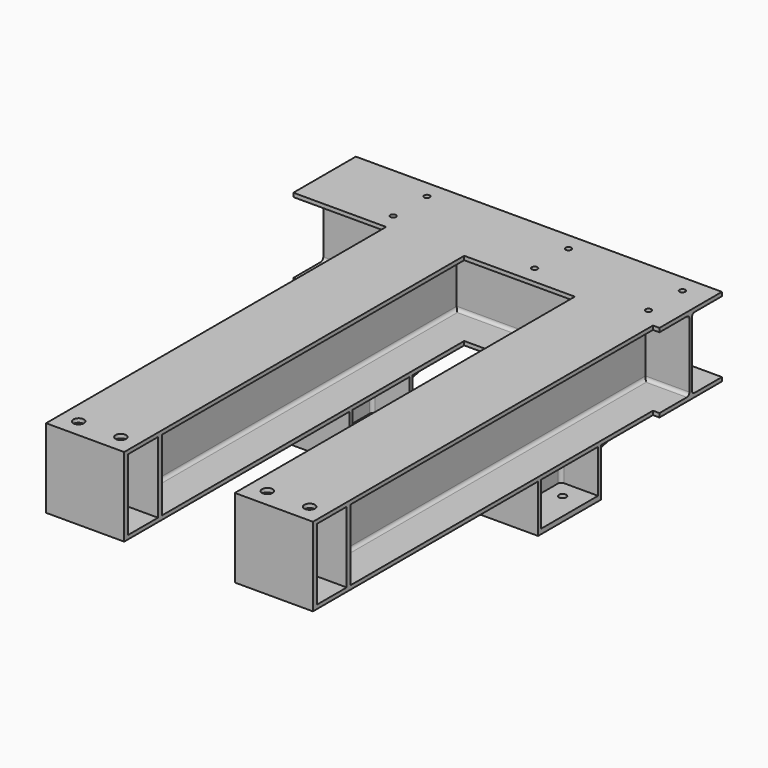
from build123d import *

# Parameters (mm, degrees)
F1_DEPTH  = 714.375
F3_D      = 22.225
F3_DEPTH  = 76.2
F3_TIP    = 6.6770636289
F5_DEPTH  = 1792.224
F6_W      = 304.8
F6_H      = 307.975
F7_DEPTH  = 19.05
F10_D     = 22.225
F10_DEPTH = 76.2
F10_TIP   = 6.6770636289
F11_W     = 19.05
F11_H     = 277.495
F12_DEPTH = 304.8
F13_W     = 19.05
F13_H     = 277.495
F14_DEPTH = 304.8
F16_D     = 41.402
F18_DEPTH = 168.402
F19_W     = 304.8
F19_H     = 307.848
F20_DEPTH = 19.05
F22_D     = 28.448
F22_2_D   = 28.448
F24_W     = 19.05
F24_H     = 457.2
F25_DEPTH = 168.402
F27_DEPTH = 1260.349


# Not quite as in the source:
# - a length typed as a fraction of an inch, garbled in the dataset ("3 / 203.2 mm" for 3/8 in), is restored


with BuildPart() as f1:
    # F0 (on Right) → F1 (new body, symmetric)
    with BuildSketch(Plane.YZ):
        with BuildLine():
            Line((152.4, 153.9875), (-152.4, 153.9875))
            Line((-152.4, 153.9875), (-152.4, 138.7475))
            Line((-152.4, 138.7475), (-19.05, 138.7475))
            ThreePointArc((-19.05, 138.7475), (-10.0697438789, 135.0277561211), (-6.35, 126.0475))
            Line((-6.35, 126.0475), (-6.35, -126.0475))
            ThreePointArc((-6.35, -126.0475), (-10.0697438789, -135.0277561211), (-19.05, -138.7475))
            Line((-19.05, -138.7475), (-152.4, -138.7475))
            Line((-152.4, -138.7475), (-152.4, -153.9875))
            Line((-152.4, -153.9875), (152.4, -153.9875))
            Line((152.4, -153.9875), (152.4, -138.7475))
            Line((152.4, -138.7475), (19.05, -138.7475))
            ThreePointArc((19.05, -138.7475), (10.0697438789, -135.0277561211), (6.35, -126.0475))
            Line((6.35, -126.0475), (6.35, 126.0475))
            ThreePointArc((6.35, 126.0475), (10.0697438789, 135.0277561211), (19.05, 138.7475))
            Line((19.05, 138.7475), (152.4, 138.7475))
            Line((152.4, 138.7475), (152.4, 153.9875))
        make_face()
    extrude(amount=F1_DEPTH, both=True)

    # F3
    with Locations(Plane.XY.offset(153.9875)):
        with Locations((-381, 82.55), (-381, -82.55), (171.45, 82.55), (171.45, -82.55), (615.95, 82.55), (615.95, -82.55)):
            Hole(F3_D / 2, depth=F3_DEPTH)
            with Locations((0, 0, -(F3_DEPTH + F3_TIP / 2))):  # 118° drill point
                Cone(0, F3_D / 2, F3_TIP, mode=Mode.SUBTRACT)


with BuildPart() as f5:
    # F4 (on Front) → F5 (new body)
    with BuildSketch(Plane.XZ):
        with BuildLine():
            Line((-47.625, 153.9875), (-352.425, 153.9875))
            Line((-352.425, 153.9875), (-352.425, 138.7475))
            Line((-352.425, 138.7475), (-219.075, 138.7475))
            ThreePointArc((-219.075, 138.7475), (-210.0947438789, 135.0277561211), (-206.375, 126.0475))
            Line((-206.375, 126.0475), (-206.375, -126.0475))
            ThreePointArc((-206.375, -126.0475), (-210.0947438789, -135.0277561211), (-219.075, -138.7475))
            Line((-219.075, -138.7475), (-352.425, -138.7475))
            Line((-352.425, -138.7475), (-352.425, -153.9875))
            Line((-352.425, -153.9875), (-47.625, -153.9875))
            Line((-47.625, -153.9875), (-47.625, -138.7475))
            Line((-47.625, -138.7475), (-180.975, -138.7475))
            ThreePointArc((-180.975, -138.7475), (-189.9552561211, -135.0277561211), (-193.675, -126.0475))
            Line((-193.675, -126.0475), (-193.675, 126.0475))
            ThreePointArc((-193.675, 126.0475), (-189.9552561211, 135.0277561211), (-180.975, 138.7475))
            Line((-180.975, 138.7475), (-47.625, 138.7475))
            Line((-47.625, 138.7475), (-47.625, 153.9875))
        make_face()
    extrude(amount=F5_DEPTH)


with BuildPart() as f5b:
    # F4 (on Front) → F5, piece 2 (new body)
    with BuildSketch(Plane.XZ):
        with BuildLine():
            Line((688.975, 153.9875), (384.175, 153.9875))
            Line((384.175, 153.9875), (384.175, 138.7475))
            Line((384.175, 138.7475), (517.525, 138.7475))
            ThreePointArc((517.525, 138.7475), (526.5052561211, 135.0277561211), (530.225, 126.0475))
            Line((530.225, 126.0475), (530.225, -126.0475))
            ThreePointArc((530.225, -126.0475), (526.5052561211, -135.0277561211), (517.525, -138.7475))
            Line((517.525, -138.7475), (384.175, -138.7475))
            Line((384.175, -138.7475), (384.175, -153.9875))
            Line((384.175, -153.9875), (688.975, -153.9875))
            Line((688.975, -153.9875), (688.975, -138.7475))
            Line((688.975, -138.7475), (555.625, -138.7475))
            ThreePointArc((555.625, -138.7475), (546.6447438789, -135.0277561211), (542.925, -126.0475))
            Line((542.925, -126.0475), (542.925, 126.0475))
            ThreePointArc((542.925, 126.0475), (546.6447438789, 135.0277561211), (555.625, 138.7475))
            Line((555.625, 138.7475), (688.975, 138.7475))
            Line((688.975, 138.7475), (688.975, 153.9875))
        make_face()
    extrude(amount=F5_DEPTH)


with BuildPart() as f7:
    # F6 (on face) → F7 (new body)
    with BuildSketch(Plane.XZ.offset(1792.224)):
        with Locations((-200.025, 0)):
            Rectangle(F6_W, F6_H)
    extrude(amount=F7_DEPTH)


with BuildPart() as f7b:
    # F6 (on face) → F7, piece 2 (new body)
    with BuildSketch(Plane.XZ.offset(1792.224)):
        with Locations((536.575, 0)):
            Rectangle(F6_W, F6_H)
    extrude(amount=F7_DEPTH)


with BuildPart() as f1_1:
    add(f1.part)

    # F8: union F5, F5b, F7b, F7
    add(f5.part)
    add(f5b.part)
    add(f7b.part)
    add(f7.part)

    # F10
    with Locations(Plane.XY.offset(153.9875)):
        with Locations((615.95, -82.55)):
            Hole(F10_D / 2, depth=F10_DEPTH)
            with Locations((0, 0, -(F10_DEPTH + F10_TIP / 2))):  # 118° drill point
                Cone(0, F10_D / 2, F10_TIP, mode=Mode.SUBTRACT)

    # F11 (on face) → F12 (join)
    with BuildSketch(Plane.YZ.offset(688.975)):
        with Locations((-1636.649, 0)):
            Rectangle(F11_W, F11_H)
    extrude(amount=-F12_DEPTH)

    # F13 (on face) → F14 (join)
    with BuildSketch(Plane(origin=(-352.425, 0, 0), x_dir=(0, -1, 0), z_dir=(-1, 0, 0))):
        with Locations((1636.649, 0)):
            Rectangle(F13_W, F13_H)
    extrude(amount=-F14_DEPTH)

    # F16 (through all)
    with Locations(Plane.XY.offset(153.9875)):
        with Locations((619.125, -1739.9), (454.025, -1739.9), (-117.475, -1739.9), (-282.575, -1739.9)):
            Hole(F16_D / 2)


with BuildPart() as f18:
    # F17 (on face) → F18 (new body)
    with BuildSketch(Plane(origin=(0, 0, -153.9875), x_dir=(1, 0, 0), z_dir=(0, 0, -1))):
        with BuildLine():
            Line((-352.425, 420.116), (-352.425, 404.876))
            Line((-352.425, 404.876), (-47.625, 404.876))
            Line((-47.625, 404.876), (-47.625, 420.116))
            Line((-47.625, 420.116), (-180.975, 420.116))
            ThreePointArc((-180.975, 420.116), (-189.9552561211, 423.8357438789), (-193.675, 432.816))
            Line((-193.675, 432.816), (-193.675, 684.784))
            ThreePointArc((-193.675, 684.784), (-189.9552561211, 693.7642561211), (-180.975, 697.484))
            Line((-180.975, 697.484), (-47.625, 697.484))
            Line((-47.625, 697.484), (-47.625, 712.724))
            Line((-47.625, 712.724), (-352.425, 712.724))
            Line((-352.425, 712.724), (-352.425, 697.484))
            Line((-352.425, 697.484), (-219.075, 697.484))
            ThreePointArc((-219.075, 697.484), (-210.0947438789, 693.7642561211), (-206.375, 684.784))
            Line((-206.375, 684.784), (-206.375, 432.816))
            ThreePointArc((-206.375, 432.816), (-210.0947438789, 423.8357438789), (-219.075, 420.116))
            Line((-219.075, 420.116), (-352.425, 420.116))
        make_face()
    extrude(amount=F18_DEPTH)


with BuildPart() as f18b:
    # F17 (on face) → F18, piece 2 (new body)
    with BuildSketch(Plane(origin=(0, 0, -153.9875), x_dir=(1, 0, 0), z_dir=(0, 0, -1))):
        with BuildLine():
            Line((688.975, 420.116), (555.625, 420.116))
            ThreePointArc((555.625, 420.116), (546.6447438789, 423.8357438789), (542.925, 432.816))
            Line((542.925, 432.816), (542.925, 684.784))
            ThreePointArc((542.925, 684.784), (546.6447438789, 693.7642561211), (555.625, 697.484))
            Line((555.625, 697.484), (688.975, 697.484))
            Line((688.975, 697.484), (688.975, 712.724))
            Line((688.975, 712.724), (384.175, 712.724))
            Line((384.175, 712.724), (384.175, 697.484))
            Line((384.175, 697.484), (517.525, 697.484))
            ThreePointArc((517.525, 697.484), (526.5052561211, 693.7642561211), (530.225, 684.784))
            Line((530.225, 684.784), (530.225, 432.816))
            ThreePointArc((530.225, 432.816), (526.5052561211, 423.8357438789), (517.525, 420.116))
            Line((517.525, 420.116), (384.175, 420.116))
            Line((384.175, 420.116), (384.175, 404.876))
            Line((384.175, 404.876), (688.975, 404.876))
            Line((688.975, 404.876), (688.975, 420.116))
        make_face()
    extrude(amount=F18_DEPTH)


with BuildPart() as f20:
    # F19 (on face) → F20 (new body)
    with BuildSketch(Plane(origin=(0, 0, -322.3895), x_dir=(1, 0, 0), z_dir=(0, 0, -1))):
        with Locations((-200.025, 558.8)):
            Rectangle(F19_W, F19_H)
    extrude(amount=F20_DEPTH)

    # F22 (through all)
    with Locations(Plane(origin=(0, 0, -341.4395), x_dir=(1, 0, 0), z_dir=(0, 0, -1))):
        with Locations((-269.1834158416, 628.65), (-130.8665841584, 628.65), (-269.1834158416, 488.95), (-130.8665841584, 488.95), (467.4165841584, 628.65), (605.7334158416, 628.65), (605.7334158416, 488.95), (467.4165841584, 488.95)):
            Hole(F22_D / 2)


with BuildPart() as f20b:
    # F19 (on face) → F20, piece 2 (new body)
    with BuildSketch(Plane(origin=(0, 0, -322.3895), x_dir=(1, 0, 0), z_dir=(0, 0, -1))):
        with Locations((536.575, 558.8)):
            Rectangle(F19_W, F19_H)
    extrude(amount=F20_DEPTH)

    # F22#2 (through all)
    with Locations(Plane(origin=(0, 0, -341.4395), x_dir=(1, 0, 0), z_dir=(0, 0, -1))):
        with Locations((-269.1834158416, 628.65), (-130.8665841584, 628.65), (-269.1834158416, 488.95), (-130.8665841584, 488.95), (467.4165841584, 628.65), (605.7334158416, 628.65), (605.7334158416, 488.95), (467.4165841584, 488.95)):
            Hole(F22_2_D / 2)


with BuildPart() as f1_2:
    add(f1_1.part)

    # F23: union F18, F20, F18b, F20b
    add(f18.part)
    add(f20.part)
    add(f18b.part)
    add(f20b.part)

    # F24 (on face) → F25 (join)
    with BuildSketch(Plane(origin=(0, 0, -153.9875), x_dir=(1, 0, 0), z_dir=(0, 0, -1))):
        with Locations((-200.152, 176.276)):
            Rectangle(F24_W, F24_H)
        with Locations((536.448, 176.276)):
            Rectangle(F24_W, F24_H)
    extrude(amount=F25_DEPTH)

    # F26 (on face) → F27 (cut, through all)
    with BuildSketch(Plane.YZ.offset(545.973)):
        Polygon((52.324, -322.3895), (52.324, -217.4875), (-404.876, -322.3895), align=None)
    extrude(amount=-F27_DEPTH, mode=Mode.SUBTRACT)


solid = f1_2.part
